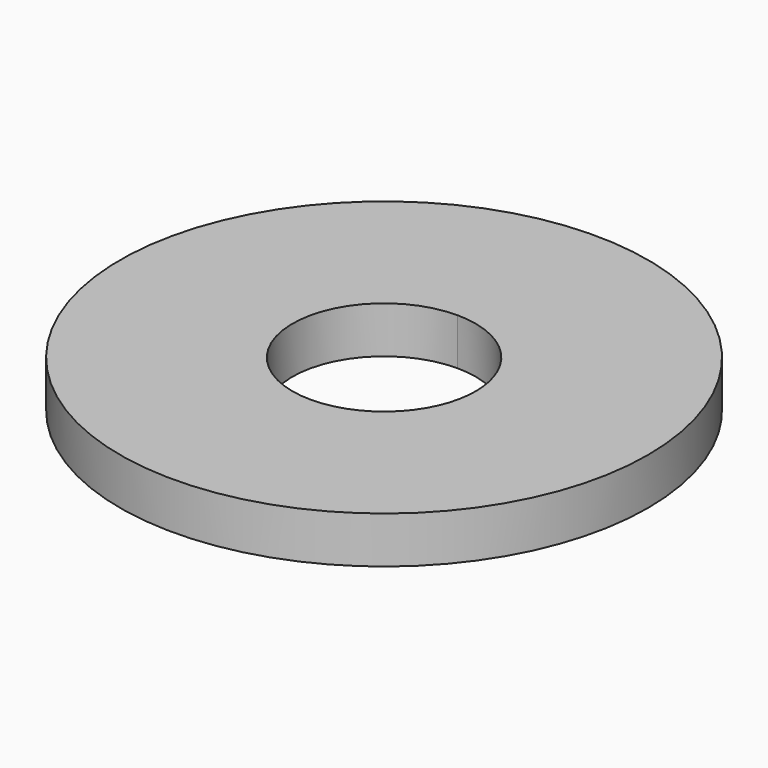
from build123d import *

# Parameters (mm, degrees)
F0_R     = 18.669
F1_DEPTH = 3.302


# Not quite as in the source:
# - a length typed as a fraction of an inch, garbled in the dataset ("3 / 203.2 mm" for 3/8 in), is restored


with BuildPart() as f1:
    # F0 (on Top) → F1 (new body)
    with BuildSketch(Plane.XY):
        Circle(F0_R)
        Polygon((-5.6092465283, 3.2385000208), (-3.7394976935, 6.477), (0, 6.477), (3.7394976935, 6.477), (5.6092465069, 3.238500058), (7.4789953871, 0), (5.6092465631, -3.2384999606), (3.7394976935, -6.477), (0, -6.477), (-3.7394976935, -6.477), (-5.6092464752, -3.2385001127), (-7.4789953871, 0), align=None, mode=Mode.SUBTRACT)
        with BuildLine():
            Line((0, 6.477), (-3.7394976935, 6.477))
            Line((-3.7394976935, 6.477), (-5.6092465283, 3.2385000208))
            ThreePointArc((-5.6092465283, 3.2385000208), (-3.2384999896, 5.6092465463), (0, 6.477))
        make_face()
        with BuildLine():
            Line((3.7394976935, 6.477), (0, 6.477))
            ThreePointArc((0, 6.477), (3.238499971, 5.609246557), (5.6092465069, 3.238500058))
            Line((5.6092465069, 3.238500058), (3.7394976935, 6.477))
        make_face()
        with BuildLine():
            ThreePointArc((5.6092465631, -3.2384999606), (3.2385000197, -5.6092465289), (0, -6.477))
            Line((0, -6.477), (3.7394976935, -6.477))
            Line((3.7394976935, -6.477), (5.6092465631, -3.2384999606))
        make_face()
        with BuildLine():
            Line((7.4789953871, 0), (5.6092465069, 3.238500058))
            ThreePointArc((5.6092465069, 3.238500058), (6.2563015682, 1.6763709874), (6.477, 0))
            ThreePointArc((6.477, 0), (6.2563015828, -1.6763709332), (5.6092465631, -3.2384999606))
            Line((5.6092465631, -3.2384999606), (7.4789953871, 0))
        make_face()
        with BuildLine():
            ThreePointArc((0, -6.477), (-3.2384999437, -5.6092465728), (-5.6092464752, -3.2385001127))
            Line((-5.6092464752, -3.2385001127), (-3.7394976935, -6.477))
            Line((-3.7394976935, -6.477), (0, -6.477))
        make_face()
        with BuildLine():
            ThreePointArc((-5.6092464752, -3.2385001127), (-6.477, -5.31e-08), (-5.6092465283, 3.2385000208))
            Line((-5.6092465283, 3.2385000208), (-7.4789953871, 0))
            Line((-7.4789953871, 0), (-5.6092464752, -3.2385001127))
        make_face()
    extrude(amount=F1_DEPTH)


solid = f1.part
